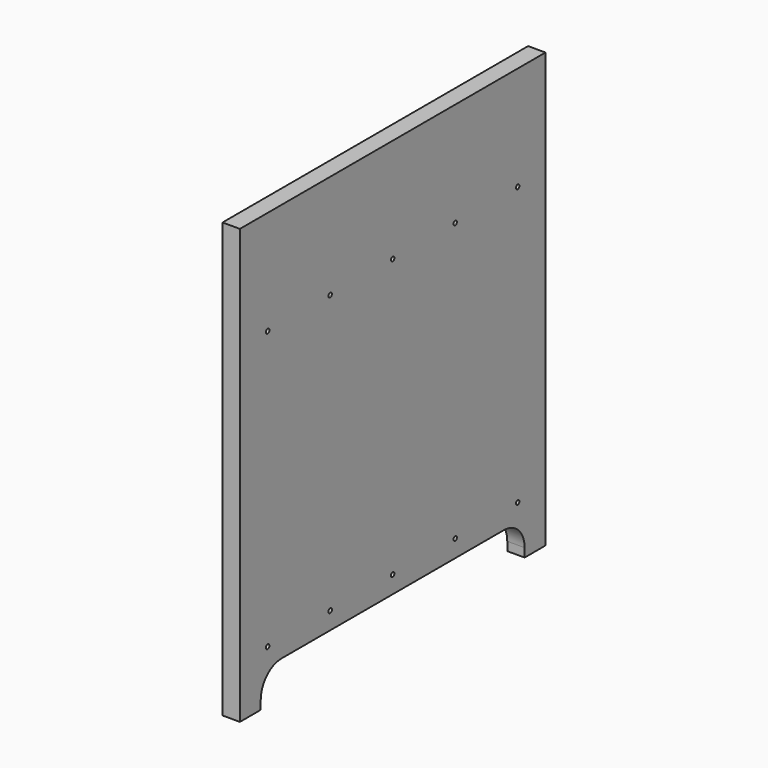
from build123d import *

# Parameters (mm, degrees)
F0_W     = 440
F0_H     = 500
F1_DEPTH = 20
F2_W     = 190
F2_H     = 40
F3_DEPTH = 20
F4_R     = 30
F6_D     = 5


# Not quite as in the source:
# - a feature names something its author has since deleted; it is built from what else it names


with BuildPart() as f1:
    # F0 (on Right) → F1 (new body)
    with BuildSketch(Plane.YZ):
        with Locations((31.3553263247, 6.565798074)):
            Rectangle(F0_W, F0_H)
    extrude(amount=F1_DEPTH)

    # F2 (on face) → F3 (cut, through all)
    with BuildSketch(Plane.YZ.offset(20)):
        with Locations((-63.6446736753, -223.434201926)):
            Rectangle(F2_W, F2_H)
        with Locations((126.3553263247, -223.434201926)):
            Rectangle(F2_W, F2_H)
    extrude(amount=-F3_DEPTH, mode=Mode.SUBTRACT)

    # F4
    f4_edges = [f1.edges().sort_by_distance(p)[0] for p in [
        (10, -158.644674, -203.434202),
        (10, 221.355326, -203.434202),
    ]]
    fillet(f4_edges, radius=F4_R)

    # F6 (through all)
    with Locations(Plane(origin=(0, 0, 0), x_dir=(0, -1, 0), z_dir=(-1, 0, 0))):
        with Locations((148.6446736753, -183.434201926), (58.6446736753, -183.434201926), (-31.3553263247, -183.434201926), (-121.3553263247, -183.434201926), (-211.3553263247, -183.434201926), (148.6446736753, 136.565798074), (58.6446736753, 136.565798074), (-31.3553263247, 136.565798074), (-121.3553263247, 136.565798074), (-211.3553263247, 136.565798074)):
            Hole(F6_D / 2)


solid = f1.part
